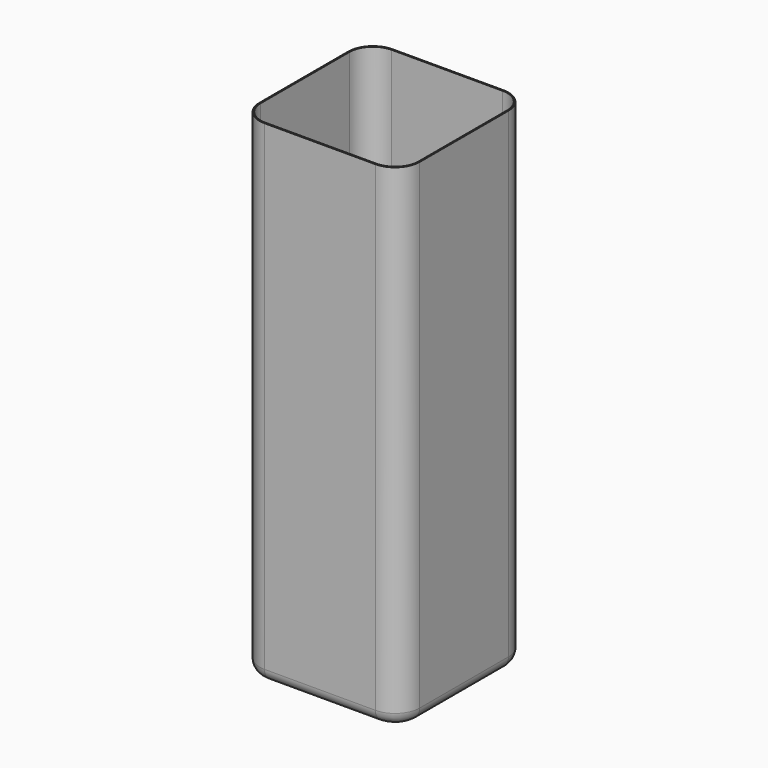
from build123d import *

# Parameters (mm, degrees)
F1_DEPTH     = 1016
F2_R         = 25.4
F3_T1_DEPTH  = 1143
F3_T4_ANGLE  = 90
F3_T6_ANGLE  = 90
F3_T8_ANGLE  = 90
F3_T10_ANGLE = 90
F4_T         = -2.54


# Not quite as in the source:
# - a fillet or chamfer that OpenCascade refuses, or shapes differently, is made with other operations: its cross-section is extruded or revolved along the edge and cut away or added


with BuildPart() as f1:
    # F0 (on Top) → F1 (new body)
    with BuildSketch(Plane.XY):
        Polygon((165.1, -165.1), (165.1, 0), (165.1, 165.1), (-165.1, 165.1), (-165.1, -165.1), align=None)
    extrude(amount=F1_DEPTH)

    # F2
    f2_edges = [f1.edges().sort_by_distance(p)[0] for p in [
        (-165.1, 0, 0),
        (0, 165.1, 0),
        (0, -165.1, 0),
        (165.1, 0, 0),
    ]]
    fillet(f2_edges, radius=F2_R)

    # F3: fillet of radius 50.8 on 4 edges, made by hand

    # F3_s2 → F3_t1 (cut)
    with BuildSketch(Plane.XY):
        with BuildLine():
            ThreePointArc((-114.3, 165.1), (-150.2210244843, 150.2210244843), (-165.1, 114.3))
            Line((-165.1, 114.3), (-165.1, 165.1))
            Line((-165.1, 165.1), (-114.3, 165.1))
        make_face()
        with BuildLine():
            ThreePointArc((-114.3, -165.1), (-150.2210244843, -150.2210244843), (-165.1, -114.3))
            Line((-165.1, -114.3), (-165.1, -165.1))
            Line((-165.1, -165.1), (-114.3, -165.1))
        make_face()
        with BuildLine():
            ThreePointArc((165.1, 114.3), (150.2210244843, 150.2210244843), (114.3, 165.1))
            Line((114.3, 165.1), (165.1, 165.1))
            Line((165.1, 165.1), (165.1, 114.3))
        make_face()
        with BuildLine():
            ThreePointArc((165.1, -114.3), (150.2210244843, -150.2210244843), (114.3, -165.1))
            Line((114.3, -165.1), (165.1, -165.1))
            Line((165.1, -165.1), (165.1, -114.3))
        make_face()
    extrude(amount=F3_T1_DEPTH, mode=Mode.SUBTRACT)

    # F3_s3 → F3_t4 (revolve, cut)
    with BuildSketch(Plane.XZ.offset(114.3)):
        with BuildLine():
            ThreePointArc((139.7, 0), (157.6605122421, 7.4394877579), (165.1, 25.4))
            Line((165.1, 25.4), (165.1, 0))
            Line((165.1, 0), (139.7, 0))
        make_face()
    revolve(axis=Axis((114.3, -114.3, 0), (0, 0, -1)), revolution_arc=F3_T4_ANGLE, mode=Mode.SUBTRACT)

    # F3_s5 → F3_t6 (revolve, cut)
    with BuildSketch(Plane.YZ.offset(114.3)):
        with BuildLine():
            ThreePointArc((139.7, 0), (157.6605122421, 7.4394877579), (165.1, 25.4))
            Line((165.1, 25.4), (165.1, 0))
            Line((165.1, 0), (139.7, 0))
        make_face()
    revolve(axis=Axis((114.3, 114.3, 0), (0, 0, -1)), revolution_arc=F3_T6_ANGLE, mode=Mode.SUBTRACT)

    # F3_s7 → F3_t8 (revolve, cut)
    with BuildSketch(Plane.YZ.offset(-114.3)):
        with BuildLine():
            ThreePointArc((-139.7, 0), (-157.6605122421, 7.4394877579), (-165.1, 25.4))
            Line((-165.1, 25.4), (-165.1, 0))
            Line((-165.1, 0), (-139.7, 0))
        make_face()
    revolve(axis=Axis((-114.3, -114.3, 0), (0, 0, -1)), revolution_arc=F3_T8_ANGLE, mode=Mode.SUBTRACT)

    # F3_s9 → F3_t10 (revolve, cut)
    with BuildSketch(Plane.XZ.offset(-114.3)):
        with BuildLine():
            ThreePointArc((-139.7, 0), (-157.6605122421, 7.4394877579), (-165.1, 25.4))
            Line((-165.1, 25.4), (-165.1, 0))
            Line((-165.1, 0), (-139.7, 0))
        make_face()
    revolve(axis=Axis((-114.3, 114.3, 0), (0, 0, -1)), revolution_arc=F3_T10_ANGLE, mode=Mode.SUBTRACT)

    # F4
    f4_openings = [f1.faces().sort_by_distance(p)[0] for p in [
        (0, 0, 1016),
    ]]
    offset(amount=F4_T, openings=f4_openings)


solid = f1.part
